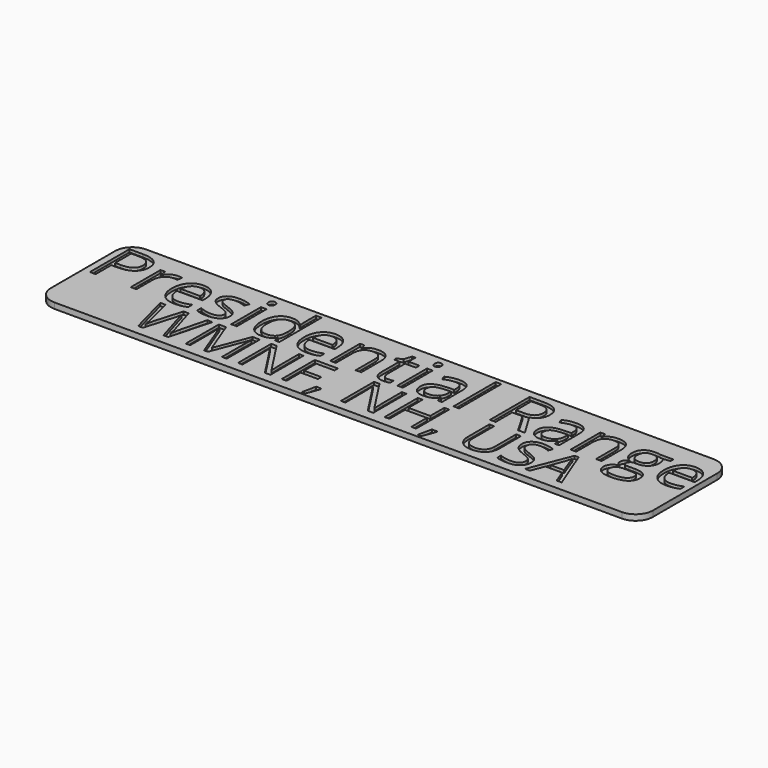
from build123d import *

# Parameters (mm, degrees)
F0_W           = 105
F0_H           = 20
F1_DEPTH       = 1
F2_TEXT_SIZE   = 12.1061449495
F2_TEXT_SIZE_2 = 10.1087964387
F3_DEPTH       = 0.5
F4_R           = 3


# Not quite as in the source:
# - Text() gives the source's letters only with a copy of the font that has no kerning and outlines rounded to 1/6400 em; it was checked with that copy


with BuildPart() as f1:
    # F0 (on Top) → F1 (new body)
    with BuildSketch(Plane.XY):
        Rectangle(F0_W, F0_H)
    extrude(amount=F1_DEPTH)

    # F2 (on face) → F3 (cut)
    with BuildSketch(Plane.XY.offset(1)):
        with Locations((-52.5, 0.011226366)):
            Text('Presidential Range', F2_TEXT_SIZE, font='Open Sans', text_align=(TextAlign.LEFT, TextAlign.BOTTOM))
        with Locations((-38.2862767619, -8.306584321)):
            Text('WMNF, NH, USA', F2_TEXT_SIZE_2, font='Open Sans', text_align=(TextAlign.LEFT, TextAlign.BOTTOM))
    extrude(amount=-F3_DEPTH, mode=Mode.SUBTRACT)

    # F4
    f4_edges = [f1.edges().sort_by_distance(p)[0] for p in [
        (-52.5, -10, 0.5),
        (-52.5, 10, 0.5),
        (52.5, 10, 0.5),
        (52.5, -10, 0.5),
    ]]
    fillet(f4_edges, radius=F4_R)


solid = f1.part
